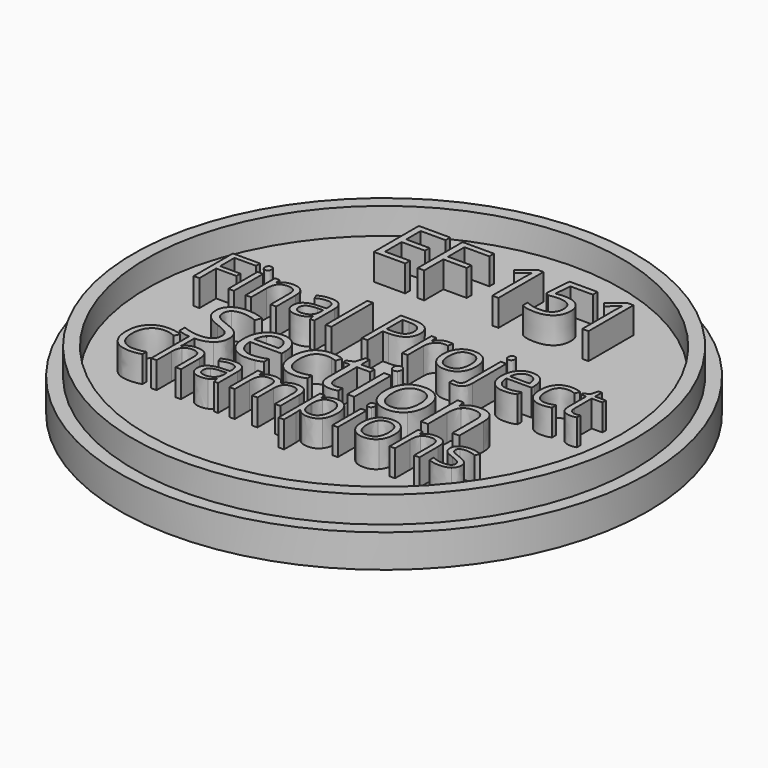
from build123d import *

# Parameters (mm, degrees)
F0_R           = 25.4
F1_DEPTH       = 3.175
F2_R           = 24.13
F2_R_2         = 22.86
F3_DEPTH       = 2.54
F4_TEXT_SIZE   = 7.5765898348
F4_TEXT_SIZE_2 = 6.592654649
F4_W           = 0.670269991
F4_H           = 4.4232653547
F4_W_2         = 0.5213210837
F4_H_2         = 3.4403173635
F5_DEPTH       = 2.54


# Not quite as in the source:
# - Text() gives the source's letters only with a copy of the font that has no kerning and outlines rounded to 1/6400 em; it was checked with that copy


with BuildPart() as f1:
    # F0 (on Top) → F1 (new body)
    with BuildSketch(Plane.XY):
        Circle(F0_R)
    extrude(amount=F1_DEPTH)

    # F2 (on face) → F3 (join)
    with BuildSketch(Plane.XY.offset(3.175)):
        Circle(F2_R)
        Circle(F2_R_2, mode=Mode.SUBTRACT)
    extrude(amount=F3_DEPTH)

    # F4 (on face) → F5 (join)
    with BuildSketch(Plane.XY.offset(3.175)):
        with Locations((-10.9458046269, 11.5243140608)):
            Text('EF 151', F4_TEXT_SIZE, font='Open Sans', text_align=(TextAlign.LEFT, TextAlign.BOTTOM))
        with Locations((-18.9641831386, 0)):
            Text('Final Project', F4_TEXT_SIZE_2, font='Open Sans', text_align=(TextAlign.LEFT, TextAlign.BOTTOM))
        with BuildLine():
            add(Edge.make_bspline(
                [(-9.8868052331, -6.2462335304), (-9.8868052331, -7.0249865257), (-10.4518208806, -7.4615014716)],
                knots=[0, 0, 0, 1, 1, 1], degree=2))
            add(Edge.make_bspline(
                [(-10.2355006041, -5.2621377055), (-9.8868052331, -5.6418282206), (-9.8868052331, -6.2462335304)],
                knots=[0, 0, 0, 1, 1, 1], degree=2))
            add(Edge.make_bspline(
                [(-11.5127588335, -4.55183232), (-10.5841959751, -4.8824471903), (-10.2355006041, -5.2621377055)],
                knots=[0, 0, 0, 1, 1, 1], degree=2))
            add(Edge.make_bspline(
                [(-12.334130152, -4.1908680378), (-12.0655055698, -4.3542382764), (-11.5127588335, -4.55183232)],
                knots=[0, 0, 0, 1, 1, 1], degree=2))
            add(Edge.make_bspline(
                [(-12.7157578636, -3.8311952199), (-12.6027547341, -4.0274977991), (-12.334130152, -4.1908680378)],
                knots=[0, 0, 0, 1, 1, 1], degree=2))
            add(Edge.make_bspline(
                [(-12.8287609931, -3.3288155927), (-12.8287609931, -3.6348926406), (-12.7157578636, -3.8311952199)],
                knots=[0, 0, 0, 1, 1, 1], degree=2))
            add(Edge.make_bspline(
                [(-12.522038213, -2.6792090312), (-12.8287609931, -2.9129640762), (-12.8287609931, -3.3288155927)],
                knots=[0, 0, 0, 1, 1, 1], degree=2))
            add(Edge.make_bspline(
                [(-11.6703174827, -2.4454539861), (-12.2153154329, -2.4454539861), (-12.522038213, -2.6792090312)],
                knots=[0, 0, 0, 1, 1, 1], degree=2))
            add(Edge.make_bspline(
                [(-10.2497067118, -2.751531034), (-10.9806755266, -2.4454539861), (-11.6703174827, -2.4454539861)],
                knots=[0, 0, 0, 1, 1, 1], degree=2))
            Line((-10.2497067118, -2.751531034), (-10.0353236318, -2.1548745103))
            add(Edge.make_bspline(
                [(-11.6535284463, -1.832008426), (-10.7740412327, -1.832008426), (-10.0353236318, -2.1548745103)],
                knots=[0, 0, 0, 1, 1, 1], degree=2))
            add(Edge.make_bspline(
                [(-13.0102117325, -2.2355910313), (-12.4981461228, -1.832008426), (-11.6535284463, -1.832008426)],
                knots=[0, 0, 0, 1, 1, 1], degree=2))
            add(Edge.make_bspline(
                [(-13.5222773421, -3.3210668067), (-13.5222773421, -2.6391736367), (-13.0102117325, -2.2355910313)],
                knots=[0, 0, 0, 1, 1, 1], degree=2))
            add(Edge.make_bspline(
                [(-13.1690618459, -4.3742559737), (-13.5222773421, -3.9706733683), (-13.5222773421, -3.3210668067)],
                knots=[0, 0, 0, 1, 1, 1], degree=2))
            add(Edge.make_bspline(
                [(-11.993183567, -5.0722924479), (-12.8158463497, -4.777838579), (-13.1690618459, -4.3742559737)],
                knots=[0, 0, 0, 1, 1, 1], degree=2))
            add(Edge.make_bspline(
                [(-11.1156335499, -5.4474628378), (-11.4042758292, -5.2815096705), (-11.993183567, -5.0722924479)],
                knots=[0, 0, 0, 1, 1, 1], degree=2))
            add(Edge.make_bspline(
                [(-10.7036564263, -5.8090728522), (-10.8269912705, -5.6134160052), (-11.1156335499, -5.4474628378)],
                knots=[0, 0, 0, 1, 1, 1], degree=2))
            add(Edge.make_bspline(
                [(-10.5803215821, -6.3108067472), (-10.5803215821, -6.0047296993), (-10.7036564263, -5.8090728522)],
                knots=[0, 0, 0, 1, 1, 1], degree=2))
            add(Edge.make_bspline(
                [(-10.9277254888, -7.0359639725), (-10.5803215821, -6.7757339086), (-10.5803215821, -6.3108067472)],
                knots=[0, 0, 0, 1, 1, 1], degree=2))
            add(Edge.make_bspline(
                [(-11.9608969585, -7.2961940365), (-11.2751293955, -7.2961940365), (-10.9277254888, -7.0359639725)],
                knots=[0, 0, 0, 1, 1, 1], degree=2))
            add(Edge.make_bspline(
                [(-12.8080975637, -7.2070829972), (-12.3806228681, -7.2961940365), (-11.9608969585, -7.2961940365)],
                knots=[0, 0, 0, 1, 1, 1], degree=2))
            add(Edge.make_bspline(
                [(-13.5997652024, -6.9655791662), (-13.2355722593, -7.1179719579), (-12.8080975637, -7.2070829972)],
                knots=[0, 0, 0, 1, 1, 1], degree=2))
            Line((-13.5997652024, -6.9655791662), (-13.5997652024, -7.6268089068))
            add(Edge.make_bspline(
                [(-12.4609801616, -7.8823944824), (-13.1698642161, -7.832925818), (-13.5997652024, -7.6268089068)],
                knots=[0.2400029386, 0.2400029386, 0.2400029386, 1, 1, 1], degree=2))
            Line((-12.4609801616, -7.8823944824), (-12.4609801616, -7.5605137475))
            Line((-12.4609801616, -7.5605137475), (-11.9396590779, -7.5605137475))
            Line((-11.9396590779, -7.5605137475), (-11.9396590779, -7.8977702507))
            add(Edge.make_bspline(
                [(-10.4518208806, -7.4615014716), (-11.0034188994, -7.887650341), (-11.9396590779, -7.8977702507)],
                knots=[0, 0, 0, 0.9762526424, 0.9762526424, 0.9762526424], degree=2))
        make_face()
        with BuildLine():
            Line((-11.9396590779, -9.0390968596), (-11.9396590779, -7.8977702507))
            add(Edge.make_bspline(
                [(-11.9396590779, -7.8977702507), (-11.9624331318, -7.8980164176), (-11.9854347809, -7.8980164176)],
                knots=[0.9762526424, 0.9762526424, 0.9762526424, 1, 1, 1], degree=2))
            add(Edge.make_bspline(
                [(-11.9854347809, -7.8980164176), (-12.2371184326, -7.8980164176), (-12.4609801616, -7.8823944824)],
                knots=[0, 0, 0, 0.2400029386, 0.2400029386, 0.2400029386], degree=2))
            Line((-12.4609801616, -7.8823944824), (-12.4609801616, -12.4452621676))
            Line((-12.4609801616, -12.4452621676), (-11.9396590779, -12.4452621676))
            Line((-11.9396590779, -12.4452621676), (-11.9396590779, -10.6462524163))
            add(Edge.make_bspline(
                [(-11.6900477305, -9.6799501379), (-11.9396590779, -9.9752649714), (-11.9396590779, -10.6462524163)],
                knots=[0, 0, 0, 1, 1, 1], degree=2))
            add(Edge.make_bspline(
                [(-10.8980213827, -9.3846353043), (-11.4404363831, -9.3846353043), (-11.6900477305, -9.6799501379)],
                knots=[0, 0, 0, 1, 1, 1], degree=2))
            add(Edge.make_bspline(
                [(-10.2978492295, -9.5920588184), (-10.4892011879, -9.3846353043), (-10.8980213827, -9.3846353043)],
                knots=[0, 0, 0, 1, 1, 1], degree=2))
            add(Edge.make_bspline(
                [(-10.106497271, -10.2193517216), (-10.106497271, -9.7994823324), (-10.2978492295, -9.5920588184)],
                knots=[0, 0, 0, 1, 1, 1], degree=2))
            Line((-10.106497271, -10.2193517216), (-10.106497271, -12.4452621676))
            Line((-10.106497271, -12.4452621676), (-9.5851761873, -12.4452621676))
            Line((-9.5851761873, -12.4452621676), (-9.5851761873, -10.2012712216))
            add(Edge.make_bspline(
                [(-9.9010827014, -9.2485293181), (-9.5851761873, -9.5483642767), (-9.5851761873, -10.2012712216)],
                knots=[0, 0, 0, 1, 1, 1], degree=2))
            add(Edge.make_bspline(
                [(-10.8477977715, -8.9486943596), (-10.2169892155, -8.9486943596), (-9.9010827014, -9.2485293181)],
                knots=[0, 0, 0, 1, 1, 1], degree=2))
            add(Edge.make_bspline(
                [(-11.4956823553, -9.0913294152), (-11.2114167162, -8.9486943596), (-10.8477977715, -8.9486943596)],
                knots=[0, 0, 0, 1, 1, 1], degree=2))
            add(Edge.make_bspline(
                [(-11.9336322445, -9.48206911), (-11.7799479944, -9.2339644709), (-11.4956823553, -9.0913294152)],
                knots=[0, 0, 0, 1, 1, 1], degree=2))
            Line((-11.9336322445, -9.48206911), (-11.9647708834, -9.48206911))
            add(Edge.make_bspline(
                [(-11.9396590779, -9.0390968596), (-11.9396590779, -9.3062864709), (-11.9647708834, -9.48206911)],
                knots=[0, 0, 0, 1, 1, 1], degree=2))
        make_face()
        with BuildLine():
            add(Edge.make_bspline(
                [(-11.9396590779, -7.8977702507), (-11.9624331318, -7.8980164176), (-11.9854347809, -7.8980164176)],
                knots=[0.9762526424, 0.9762526424, 0.9762526424, 1, 1, 1], degree=2))
            Line((-11.9396590779, -7.8977702507), (-11.9396590779, -7.5605137475))
            Line((-11.9396590779, -7.5605137475), (-12.4609801616, -7.5605137475))
            Line((-12.4609801616, -7.5605137475), (-12.4609801616, -7.8823944824))
            add(Edge.make_bspline(
                [(-11.9854347809, -7.8980164176), (-12.2371184326, -7.8980164176), (-12.4609801616, -7.8823944824)],
                knots=[0, 0, 0, 0.2400029386, 0.2400029386, 0.2400029386], degree=2))
        make_face()
        with BuildLine():
            add(Edge.make_bspline(
                [(-6.9112714003, -7.8980164176), (-7.8914928322, -7.8980164176), (-8.4590914083, -7.3000684295)],
                knots=[0, 0, 0, 1, 1, 1], degree=2))
            add(Edge.make_bspline(
                [(-6.1467245127, -7.8308602721), (-6.4631332753, -7.8980164176), (-6.9112714003, -7.8980164176)],
                knots=[0, 0, 0, 1, 1, 1], degree=2))
            add(Edge.make_bspline(
                [(-5.4751630574, -7.6113113347), (-5.8303157501, -7.7637041265), (-6.1467245127, -7.8308602721)],
                knots=[0, 0, 0, 1, 1, 1], degree=2))
            Line((-5.4751630574, -7.6113113347), (-5.4751630574, -7.0133633466))
            add(Edge.make_bspline(
                [(-6.8867335779, -7.3116916085), (-6.1725537994, -7.3116916085), (-5.4751630574, -7.0133633466)],
                knots=[0, 0, 0, 1, 1, 1], degree=2))
            add(Edge.make_bspline(
                [(-7.9379855483, -6.9081090032), (-7.5647523549, -7.3116916085), (-6.8867335779, -7.3116916085)],
                knots=[0, 0, 0, 1, 1, 1], degree=2))
            add(Edge.make_bspline(
                [(-8.3318821711, -5.7257734025), (-8.3112187417, -6.5045263978), (-7.9379855483, -6.9081090032)],
                knots=[0, 0, 0, 1, 1, 1], degree=2))
            Line((-8.3318821711, -5.7257734025), (-5.2853177998, -5.7257734025))
            Line((-5.2853177998, -5.7257734025), (-5.2853177998, -5.3021730999))
            add(Edge.make_bspline(
                [(-5.7696169262, -3.8589617031), (-5.2853177998, -4.4058968499), (-5.2853177998, -5.3021730999)],
                knots=[0, 0, 0, 1, 1, 1], degree=2))
            add(Edge.make_bspline(
                [(-7.0843276214, -3.3120265564), (-6.2539160527, -3.3120265564), (-5.7696169262, -3.8589617031)],
                knots=[0, 0, 0, 1, 1, 1], degree=2))
            add(Edge.make_bspline(
                [(-8.499772535, -3.9416154207), (-7.9728550854, -3.3120265564), (-7.0843276214, -3.3120265564)],
                knots=[0, 0, 0, 1, 1, 1], degree=2))
            add(Edge.make_bspline(
                [(-9.0266899845, -5.6418282206), (-9.0266899845, -4.5712042851), (-8.499772535, -3.9416154207)],
                knots=[0, 0, 0, 1, 1, 1], degree=2))
            add(Edge.make_bspline(
                [(-8.4590914083, -7.3000684295), (-9.0266899845, -6.7021204414), (-9.0266899845, -5.6418282206)],
                knots=[0, 0, 0, 1, 1, 1], degree=2))
        make_face()
        with BuildLine():
            add(Edge.make_bspline(
                [(-7.0933678718, -3.873813543), (-7.6254511787, -3.873813543), (-7.9425056735, -4.2205717175)],
                knots=[0, 0, 0, 1, 1, 1], degree=2))
            add(Edge.make_bspline(
                [(-6.2855569289, -4.210885735), (-6.5677418866, -3.873813543), (-7.0933678718, -3.873813543)],
                knots=[0, 0, 0, 1, 1, 1], degree=2))
            add(Edge.make_bspline(
                [(-6.0033719712, -5.1807754522), (-6.0033719712, -4.547957927), (-6.2855569289, -4.210885735)],
                knots=[0, 0, 0, 1, 1, 1], degree=2))
            Line((-6.0033719712, -5.1807754522), (-8.3163845991, -5.1807754522))
            add(Edge.make_bspline(
                [(-7.9425056735, -4.2205717175), (-8.2595601682, -4.5673298921), (-8.3163845991, -5.1807754522)],
                knots=[0, 0, 0, 1, 1, 1], degree=2))
        make_face(mode=Mode.SUBTRACT)
        with BuildLine():
            add(Edge.make_bspline(
                [(-2.3743571839, -7.8980164176), (-3.3352066507, -7.8980164176), (-3.8621241003, -7.3065257512)],
                knots=[0, 0, 0, 1, 1, 1], degree=2))
            add(Edge.make_bspline(
                [(-1.2572405322, -7.6668443012), (-1.7002127999, -7.8980164176), (-2.3743571839, -7.8980164176)],
                knots=[0, 0, 0, 1, 1, 1], degree=2))
            Line((-1.2572405322, -7.6668443012), (-1.2572405322, -7.0740621705))
            add(Edge.make_bspline(
                [(-2.3911462202, -7.3116916085), (-1.8383994839, -7.3116916085), (-1.2572405322, -7.0740621705)],
                knots=[0, 0, 0, 1, 1, 1], degree=2))
            add(Edge.make_bspline(
                [(-3.3655560626, -6.8758223947), (-3.0368783888, -7.3116916085), (-2.3911462202, -7.3116916085)],
                knots=[0, 0, 0, 1, 1, 1], degree=2))
            add(Edge.make_bspline(
                [(-3.6942337364, -5.6250391842), (-3.6942337364, -6.4399531809), (-3.3655560626, -6.8758223947)],
                knots=[0, 0, 0, 1, 1, 1], degree=2))
            add(Edge.make_bspline(
                [(-2.3459449684, -3.9061001515), (-3.6942337364, -3.9061001515), (-3.6942337364, -5.6250391842)],
                knots=[0, 0, 0, 1, 1, 1], degree=2))
            add(Edge.make_bspline(
                [(-1.8823092714, -3.9642160466), (-2.1444765318, -3.9061001515), (-2.3459449684, -3.9061001515)],
                knots=[0, 0, 0, 1, 1, 1], degree=2))
            add(Edge.make_bspline(
                [(-1.398010145, -4.1114429811), (-1.620142011, -4.0223319418), (-1.8823092714, -3.9642160466)],
                knots=[0, 0, 0, 1, 1, 1], degree=2))
            Line((-1.398010145, -4.1114429811), (-1.1926673154, -3.5431986727))
            add(Edge.make_bspline(
                [(-1.6924640138, -3.3811198984), (-1.3734723226, -3.4502132404), (-1.1926673154, -3.5431986727)],
                knots=[0, 0, 0, 1, 1, 1], degree=2))
            add(Edge.make_bspline(
                [(-2.3304473964, -3.3120265564), (-2.0114557051, -3.3120265564), (-1.6924640138, -3.3811198984)],
                knots=[0, 0, 0, 1, 1, 1], degree=2))
            add(Edge.make_bspline(
                [(-3.8537295821, -3.9177233305), (-3.3184176143, -3.3120265564), (-2.3304473964, -3.3120265564)],
                knots=[0, 0, 0, 1, 1, 1], degree=2))
            add(Edge.make_bspline(
                [(-4.3890415498, -5.6327879702), (-4.3890415498, -4.5234201046), (-3.8537295821, -3.9177233305)],
                knots=[0, 0, 0, 1, 1, 1], degree=2))
            add(Edge.make_bspline(
                [(-3.8621241003, -7.3065257512), (-4.3890415498, -6.7150350848), (-4.3890415498, -5.6327879702)],
                knots=[0, 0, 0, 1, 1, 1], degree=2))
        make_face()
        with BuildLine():
            add(Edge.make_bspline(
                [(1.2210795308, -7.3439782169), (1.3993016093, -7.3439782169), (1.5646090445, -7.3181489302)],
                knots=[0, 0, 0, 1, 1, 1], degree=2))
            add(Edge.make_bspline(
                [(0.7006194029, -7.1302408691), (0.8904646605, -7.3439782169), (1.2210795308, -7.3439782169)],
                knots=[0, 0, 0, 1, 1, 1], degree=2))
            add(Edge.make_bspline(
                [(0.5107741453, -6.5174410412), (0.5107741453, -6.9165035213), (0.7006194029, -7.1302408691)],
                knots=[0, 0, 0, 1, 1, 1], degree=2))
            Line((0.5107741453, -6.5174410412), (0.5107741453, -3.9138489375))
            Line((0.5107741453, -3.9138489375), (1.7944896965, -3.9138489375))
            Line((1.7944896965, -3.9138489375), (1.7944896965, -3.3933888096))
            Line((1.7944896965, -3.3933888096), (0.5107741453, -3.3933888096))
            Line((0.5107741453, -3.3933888096), (0.5107741453, -2.3679661259))
            Line((0.5107741453, -2.3679661259), (0.1233348442, -2.3679661259))
            Line((0.1233348442, -2.3679661259), (-0.1582043813, -3.3120265564))
            Line((-0.1582043813, -3.3120265564), (-0.7923133708, -3.5909828532))
            Line((-0.7923133708, -3.5909828532), (-0.7923133708, -3.9138489375))
            Line((-0.7923133708, -3.9138489375), (-0.1582043813, -3.9138489375))
            Line((-0.1582043813, -3.9138489375), (-0.1582043813, -6.5458532566))
            add(Edge.make_bspline(
                [(1.1242197055, -7.8980164176), (-0.1582043813, -7.8980164176), (-0.1582043813, -6.5458532566)],
                knots=[0, 0, 0, 1, 1, 1], degree=2))
            add(Edge.make_bspline(
                [(1.5064931493, -7.8631468805), (1.294692998, -7.8980164176), (1.1242197055, -7.8980164176)],
                knots=[0, 0, 0, 1, 1, 1], degree=2))
            add(Edge.make_bspline(
                [(1.8267763049, -7.7766187699), (1.7182933006, -7.8282773434), (1.5064931493, -7.8631468805)],
                knots=[0, 0, 0, 1, 1, 1], degree=2))
            Line((1.8267763049, -7.7766187699), (1.8267763049, -7.263907428))
            add(Edge.make_bspline(
                [(1.5646090445, -7.3181489302), (1.7299164796, -7.2923196435), (1.8267763049, -7.263907428)],
                knots=[0, 0, 0, 1, 1, 1], degree=2))
        make_face()
        with Locations((3.045272907, -5.605021487)):
            Rectangle(F4_W, F4_H)
        with BuildLine():
            add(Edge.make_bspline(
                [(2.6533134807, -2.1949099047), (2.6533134807, -1.9650292527), (2.7663166102, -1.8578377127)],
                knots=[0, 0, 0, 1, 1, 1], degree=2))
            add(Edge.make_bspline(
                [(2.7663166102, -2.5319820967), (2.6533134807, -2.4209161637), (2.6533134807, -2.1949099047)],
                knots=[0, 0, 0, 1, 1, 1], degree=2))
            add(Edge.make_bspline(
                [(3.0497930322, -2.6430480297), (2.8793197397, -2.6430480297), (2.7663166102, -2.5319820967)],
                knots=[0, 0, 0, 1, 1, 1], degree=2))
            add(Edge.make_bspline(
                [(3.3281035968, -2.5319820967), (3.2112260743, -2.6430480297), (3.0497930322, -2.6430480297)],
                knots=[0, 0, 0, 1, 1, 1], degree=2))
            add(Edge.make_bspline(
                [(3.4449811194, -2.1949099047), (3.4449811194, -2.4209161637), (3.3281035968, -2.5319820967)],
                knots=[0, 0, 0, 1, 1, 1], degree=2))
            add(Edge.make_bspline(
                [(3.3281035968, -1.8597749092), (3.4449811194, -1.9689036457), (3.4449811194, -2.1949099047)],
                knots=[0, 0, 0, 1, 1, 1], degree=2))
            add(Edge.make_bspline(
                [(3.0497930322, -1.7506461727), (3.2112260743, -1.7506461727), (3.3281035968, -1.8597749092)],
                knots=[0, 0, 0, 1, 1, 1], degree=2))
            add(Edge.make_bspline(
                [(2.7663166102, -1.8578377127), (2.8793197397, -1.7506461727), (3.0497930322, -1.7506461727)],
                knots=[0, 0, 0, 1, 1, 1], degree=2))
        make_face()
        with BuildLine():
            add(Edge.make_bspline(
                [(8.618587254, -5.6005013618), (8.618587254, -6.6827484763), (8.0742350359, -7.290382447)],
                knots=[0, 0, 0, 1, 1, 1], degree=2))
            add(Edge.make_bspline(
                [(8.0716521072, -3.9299922417), (8.618587254, -4.547957927), (8.618587254, -5.6005013618)],
                knots=[0, 0, 0, 1, 1, 1], degree=2))
            add(Edge.make_bspline(
                [(6.5974455663, -3.3120265564), (7.5247169604, -3.3120265564), (8.0716521072, -3.9299922417)],
                knots=[0, 0, 0, 1, 1, 1], degree=2))
            add(Edge.make_bspline(
                [(5.0954725422, -3.915786134), (5.6365960995, -3.3120265564), (6.5974455663, -3.3120265564)],
                knots=[0, 0, 0, 1, 1, 1], degree=2))
            add(Edge.make_bspline(
                [(4.554348985, -5.6005013618), (4.554348985, -4.5195457116), (5.0954725422, -3.915786134)],
                knots=[0, 0, 0, 1, 1, 1], degree=2))
            add(Edge.make_bspline(
                [(4.8048930664, -6.8196436961), (4.554348985, -6.2991835682), (4.554348985, -5.6005013618)],
                knots=[0, 0, 0, 1, 1, 1], degree=2))
            add(Edge.make_bspline(
                [(5.5151984518, -7.6190601208), (5.0554371478, -7.3401038239), (4.8048930664, -6.8196436961)],
                knots=[0, 0, 0, 1, 1, 1], degree=2))
            add(Edge.make_bspline(
                [(6.5690333509, -7.8980164176), (5.9749597558, -7.8980164176), (5.5151984518, -7.6190601208)],
                knots=[0, 0, 0, 1, 1, 1], degree=2))
            add(Edge.make_bspline(
                [(8.0742350359, -7.290382447), (7.5298828178, -7.8980164176), (6.5690333509, -7.8980164176)],
                knots=[0, 0, 0, 1, 1, 1], degree=2))
        make_face()
        with BuildLine():
            add(Edge.make_bspline(
                [(5.2491567984, -5.6005013618), (5.2491567984, -6.4489934313), (5.5881661869, -6.8926114311)],
                knots=[0, 0, 0, 1, 1, 1], degree=2))
            add(Edge.make_bspline(
                [(5.5842917938, -4.3135571498), (5.2491567984, -4.7455519706), (5.2491567984, -5.6005013618)],
                knots=[0, 0, 0, 1, 1, 1], degree=2))
            add(Edge.make_bspline(
                [(6.5767821369, -3.881562329), (5.9194267893, -3.881562329), (5.5842917938, -4.3135571498)],
                knots=[0, 0, 0, 1, 1, 1], degree=2))
            add(Edge.make_bspline(
                [(7.5841243199, -4.3193687393), (7.2431777349, -3.881562329), (6.5767821369, -3.881562329)],
                knots=[0, 0, 0, 1, 1, 1], degree=2))
            add(Edge.make_bspline(
                [(7.9250709049, -5.6005013618), (7.9250709049, -4.7571751496), (7.5841243199, -4.3193687393)],
                knots=[0, 0, 0, 1, 1, 1], degree=2))
            add(Edge.make_bspline(
                [(7.5841243199, -6.8945486276), (7.9250709049, -6.4528678243), (7.9250709049, -5.6005013618)],
                knots=[0, 0, 0, 1, 1, 1], degree=2))
            add(Edge.make_bspline(
                [(6.584530923, -7.3362294309), (7.2431777349, -7.3362294309), (7.5841243199, -6.8945486276)],
                knots=[0, 0, 0, 1, 1, 1], degree=2))
            add(Edge.make_bspline(
                [(5.5881661869, -6.8926114311), (5.9271755754, -7.3362294309), (6.584530923, -7.3362294309)],
                knots=[0, 0, 0, 1, 1, 1], degree=2))
        make_face(mode=Mode.SUBTRACT)
        with BuildLine():
            Line((12.8210122071, -4.9547691932), (12.8210122071, -7.8166541643))
            Line((12.8210122071, -7.8166541643), (13.491282198, -7.8166541643))
            Line((13.491282198, -7.8166541643), (13.491282198, -4.9315228351))
            add(Edge.make_bspline(
                [(13.0876995927, -3.697528661), (13.491282198, -4.0830307656), (13.491282198, -4.9315228351)],
                knots=[0, 0, 0, 1, 1, 1], degree=2))
            add(Edge.make_bspline(
                [(11.8847005626, -3.3120265564), (12.6841169873, -3.3120265564), (13.0876995927, -3.697528661)],
                knots=[0, 0, 0, 1, 1, 1], degree=2))
            add(Edge.make_bspline(
                [(11.0575176547, -3.4921858314), (11.4288136516, -3.3120265564), (11.8847005626, -3.3120265564)],
                knots=[0, 0, 0, 1, 1, 1], degree=2))
            add(Edge.make_bspline(
                [(10.4795873638, -3.9990855837), (10.6862216578, -3.6723451064), (11.0575176547, -3.4921858314)],
                knots=[0, 0, 0, 1, 1, 1], degree=2))
            Line((10.4795873638, -3.9990855837), (10.4473007554, -3.9990855837))
            Line((10.4473007554, -3.9990855837), (10.3388177511, -3.3933888096))
            Line((10.3388177511, -3.3933888096), (9.7938198008, -3.3933888096))
            Line((9.7938198008, -3.3933888096), (9.7938198008, -7.8166541643))
            Line((9.7938198008, -7.8166541643), (10.4640897918, -7.8166541643))
            Line((10.4640897918, -7.8166541643), (10.4640897918, -5.4958927505))
            add(Edge.make_bspline(
                [(10.7869558761, -4.256732719), (10.4640897918, -4.6319031089), (10.4640897918, -5.4958927505)],
                knots=[0, 0, 0, 1, 1, 1], degree=2))
            add(Edge.make_bspline(
                [(11.8033383094, -3.881562329), (11.1098219603, -3.881562329), (10.7869558761, -4.256732719)],
                knots=[0, 0, 0, 1, 1, 1], degree=2))
            add(Edge.make_bspline(
                [(12.5749882508, -4.1482497147), (12.3289642946, -3.881562329), (11.8033383094, -3.881562329)],
                knots=[0, 0, 0, 1, 1, 1], degree=2))
            add(Edge.make_bspline(
                [(12.8210122071, -4.9547691932), (12.8210122071, -4.4149371003), (12.5749882508, -4.1482497147)],
                knots=[0, 0, 0, 1, 1, 1], degree=2))
        make_face()
        with BuildLine():
            add(Edge.make_bspline(
                [(-14.4739424963, -8.2676621924), (-15.2303100802, -8.2676621924), (-15.6682599694, -8.7714050122)],
                knots=[0, 0, 0, 1, 1, 1], degree=2))
            add(Edge.make_bspline(
                [(-13.4313003289, -8.5117489426), (-13.9526214126, -8.2676621924), (-14.4739424963, -8.2676621924)],
                knots=[0, 0, 0, 1, 1, 1], degree=2))
            Line((-13.4313003289, -8.5117489426), (-13.2052940787, -8.053709609))
            add(Edge.make_bspline(
                [(-14.4669111907, -7.7905378865), (-13.7457001347, -7.7905378865), (-13.2052940787, -8.053709609)],
                knots=[0, 0, 0, 1, 1, 1], degree=2))
            add(Edge.make_bspline(
                [(-15.6456593443, -8.0793236506), (-15.1449299412, -7.7905378865), (-14.4669111907, -7.7905378865)],
                knots=[0, 0, 0, 1, 1, 1], degree=2))
            add(Edge.make_bspline(
                [(-16.4115694143, -8.9014841651), (-16.1463887475, -8.3681094147), (-15.6456593443, -8.0793236506)],
                knots=[0, 0, 0, 1, 1, 1], degree=2))
            add(Edge.make_bspline(
                [(-16.6767500812, -10.1440163049), (-16.6767500812, -9.4348589155), (-16.4115694143, -8.9014841651)],
                knots=[0, 0, 0, 1, 1, 1], degree=2))
            add(Edge.make_bspline(
                [(-16.1257970669, -11.892802445), (-16.6767500812, -11.2770609723), (-16.6767500812, -10.1440163049)],
                knots=[0, 0, 0, 1, 1, 1], degree=2))
            add(Edge.make_bspline(
                [(-14.5613315797, -12.5085439176), (-15.5748440526, -12.5085439176), (-16.1257970669, -11.892802445)],
                knots=[0, 0, 0, 1, 1, 1], degree=2))
            add(Edge.make_bspline(
                [(-13.3840901344, -12.3287433897), (-13.8612144403, -12.5085439176), (-14.5613315797, -12.5085439176)],
                knots=[0, 0, 0, 1, 1, 1], degree=2))
            Line((-13.3840901344, -12.3287433897), (-13.3840901344, -11.8616638061))
            add(Edge.make_bspline(
                [(-14.4799693296, -12.0344330284), (-13.9998316071, -12.0344330284), (-13.3840901344, -11.8616638061)],
                knots=[0, 0, 0, 1, 1, 1], degree=2))
            add(Edge.make_bspline(
                [(-15.6838292888, -11.5427438753), (-15.2614487191, -12.0344330284), (-14.4799693296, -12.0344330284)],
                knots=[0, 0, 0, 1, 1, 1], degree=2))
            add(Edge.make_bspline(
                [(-16.1062098586, -10.1510476104), (-16.1062098586, -11.0510547222), (-15.6838292888, -11.5427438753)],
                knots=[0, 0, 0, 1, 1, 1], degree=2))
            add(Edge.make_bspline(
                [(-15.6682599694, -8.7714050122), (-16.1062098586, -9.275147832), (-16.1062098586, -10.1510476104)],
                knots=[0, 0, 0, 1, 1, 1], degree=2))
        make_face()
        with BuildLine():
            Line((-6.5034554074, -11.9550797228), (-6.3999947684, -12.4452621676))
            Line((-6.3999947684, -12.4452621676), (-6.0132729626, -12.4452621676))
            Line((-6.0132729626, -12.4452621676), (-6.0132729626, -10.0968061104))
            add(Edge.make_bspline(
                [(-6.3100945044, -9.2214085681), (-6.0132729626, -9.4941227766), (-6.0132729626, -10.0968061104)],
                knots=[0, 0, 0, 1, 1, 1], degree=2))
            add(Edge.make_bspline(
                [(-7.2216530468, -8.9486943596), (-6.6069160463, -8.9486943596), (-6.3100945044, -9.2214085681)],
                knots=[0, 0, 0, 1, 1, 1], degree=2))
            add(Edge.make_bspline(
                [(-7.8298609777, -9.027043193), (-7.5270126025, -8.9486943596), (-7.2216530468, -8.9486943596)],
                knots=[0, 0, 0, 1, 1, 1], degree=2))
            add(Edge.make_bspline(
                [(-8.3868408253, -9.2430047209), (-8.1327093529, -9.1053920264), (-7.8298609777, -9.027043193)],
                knots=[0, 0, 0, 1, 1, 1], degree=2))
            Line((-8.3868408253, -9.2430047209), (-8.2261252697, -9.6417801934))
            add(Edge.make_bspline(
                [(-7.2537961579, -9.378608471), (-7.6837102693, -9.378608471), (-8.2261252697, -9.6417801934)],
                knots=[0, 0, 0, 1, 1, 1], degree=2))
            add(Edge.make_bspline(
                [(-6.6963140742, -9.5714671378), (-6.8700877687, -9.378608471), (-7.2537961579, -9.378608471)],
                knots=[0, 0, 0, 1, 1, 1], degree=2))
            add(Edge.make_bspline(
                [(-6.5225403796, -10.1691281104), (-6.5225403796, -9.7643258046), (-6.6963140742, -9.5714671378)],
                knots=[0, 0, 0, 1, 1, 1], degree=2))
            Line((-6.5225403796, -10.1691281104), (-6.5225403796, -10.3830806939))
            Line((-6.5225403796, -10.3830806939), (-7.1061387411, -10.4021656662))
            add(Edge.make_bspline(
                [(-8.772558159, -11.4940269725), (-8.772558159, -10.4523892773), (-7.1061387411, -10.4021656662)],
                knots=[0, 0, 0, 1, 1, 1], degree=2))
            add(Edge.make_bspline(
                [(-8.4822656865, -12.244367723), (-8.772558159, -11.9801915284), (-8.772558159, -11.4940269725)],
                knots=[0, 0, 0, 1, 1, 1], degree=2))
            add(Edge.make_bspline(
                [(-7.6806968526, -12.5085439176), (-8.1919732141, -12.5085439176), (-8.4822656865, -12.244367723)],
                knots=[0, 0, 0, 1, 1, 1], degree=2))
            add(Edge.make_bspline(
                [(-7.0413502827, -12.3935318481), (-7.2969884635, -12.5085439176), (-7.6806968526, -12.5085439176)],
                knots=[0, 0, 0, 1, 1, 1], degree=2))
            add(Edge.make_bspline(
                [(-6.5285672129, -11.9550797228), (-6.785712102, -12.2785197786), (-7.0413502827, -12.3935318481)],
                knots=[0, 0, 0, 1, 1, 1], degree=2))
            Line((-6.5285672129, -11.9550797228), (-6.5034554074, -11.9550797228))
        make_face()
        with BuildLine():
            add(Edge.make_bspline(
                [(-7.5772362137, -12.077625334), (-7.0900671855, -12.077625334), (-6.8123306159, -11.8109379588)],
                knots=[0, 0, 0, 1, 1, 1], degree=2))
            add(Edge.make_bspline(
                [(-8.0553649918, -11.9304701534), (-7.8846047139, -12.077625334), (-7.5772362137, -12.077625334)],
                knots=[0, 0, 0, 1, 1, 1], degree=2))
            add(Edge.make_bspline(
                [(-8.2261252697, -11.5000538058), (-8.2261252697, -11.7833149727), (-8.0553649918, -11.9304701534)],
                knots=[0, 0, 0, 1, 1, 1], degree=2))
            add(Edge.make_bspline(
                [(-7.9519043528, -10.9681857638), (-8.2261252697, -11.1394482778), (-8.2261252697, -11.5000538058)],
                knots=[0, 0, 0, 1, 1, 1], degree=2))
            add(Edge.make_bspline(
                [(-7.05591513, -10.7748248609), (-7.677683436, -10.7969232498), (-7.9519043528, -10.9681857638)],
                knots=[0, 0, 0, 1, 1, 1], degree=2))
            Line((-7.05591513, -10.7748248609), (-6.5345940463, -10.7537309442))
            Line((-6.5345940463, -10.7537309442), (-6.5345940463, -11.0641128611))
            add(Edge.make_bspline(
                [(-6.8123306159, -11.8109379588), (-6.5345940463, -11.5442505836), (-6.5345940463, -11.0641128611)],
                knots=[0, 0, 0, 1, 1, 1], degree=2))
        make_face(mode=Mode.SUBTRACT)
        with BuildLine():
            Line((-0.5549709032, -10.2072980549), (-0.5549709032, -12.4452621676))
            Line((-0.5549709032, -12.4452621676), (-0.0346542917, -12.4452621676))
            Line((-0.0346542917, -12.4452621676), (-0.0346542917, -10.2012712216))
            add(Edge.make_bspline(
                [(-0.3249467641, -9.2414980126), (-0.0346542917, -9.5413329711), (-0.0346542917, -10.2012712216)],
                knots=[0, 0, 0, 1, 1, 1], degree=2))
            add(Edge.make_bspline(
                [(-1.1988375981, -8.941663054), (-0.6152392365, -8.941663054), (-0.3249467641, -9.2414980126)],
                knots=[0, 0, 0, 1, 1, 1], degree=2))
            add(Edge.make_bspline(
                [(-1.8643004458, -9.0988629569), (-1.572501265, -8.941663054), (-1.1988375981, -8.941663054)],
                knots=[0, 0, 0, 1, 1, 1], degree=2))
            add(Edge.make_bspline(
                [(-2.3097838766, -9.5262658878), (-2.1560996265, -9.2560628598), (-1.8643004458, -9.0988629569)],
                knots=[0, 0, 0, 1, 1, 1], degree=2))
            Line((-2.3097838766, -9.5262658878), (-2.3348956822, -9.5262658878))
            add(Edge.make_bspline(
                [(-3.3895915163, -8.941663054), (-2.5830003213, -8.941663054), (-2.3348956822, -9.5262658878)],
                knots=[0, 0, 0, 1, 1, 1], degree=2))
            add(Edge.make_bspline(
                [(-3.9907681417, -9.0832936375), (-3.7220718221, -8.941663054), (-3.3895915163, -8.941663054)],
                knots=[0, 0, 0, 1, 1, 1], degree=2))
            add(Edge.make_bspline(
                [(-4.4071218781, -9.4760422766), (-4.2594644613, -9.2249242209), (-3.9907681417, -9.0832936375)],
                knots=[0, 0, 0, 1, 1, 1], degree=2))
            Line((-4.4071218781, -9.4760422766), (-4.4322336837, -9.4760422766))
            Line((-4.4322336837, -9.4760422766), (-4.5166093504, -9.0049448041))
            Line((-4.5166093504, -9.0049448041), (-4.9404966285, -9.0049448041))
            Line((-4.9404966285, -9.0049448041), (-4.9404966285, -12.4452621676))
            Line((-4.9404966285, -12.4452621676), (-4.4191755448, -12.4452621676))
            Line((-4.4191755448, -12.4452621676), (-4.4191755448, -10.640225583))
            add(Edge.make_bspline(
                [(-4.1916625863, -9.6779411934), (-4.4191755448, -9.9712470825), (-4.4191755448, -10.640225583)],
                knots=[0, 0, 0, 1, 1, 1], degree=2))
            add(Edge.make_bspline(
                [(-3.4749716552, -9.3846353043), (-3.9641496278, -9.3846353043), (-4.1916625863, -9.6779411934)],
                knots=[0, 0, 0, 1, 1, 1], degree=2))
            add(Edge.make_bspline(
                [(-2.9255253493, -9.5900498739), (-3.1013079883, -9.3846353043), (-3.4749716552, -9.3846353043)],
                knots=[0, 0, 0, 1, 1, 1], degree=2))
            add(Edge.make_bspline(
                [(-2.7497427103, -10.2072980549), (-2.7497427103, -9.7954644435), (-2.9255253493, -9.5900498739)],
                knots=[0, 0, 0, 1, 1, 1], degree=2))
            Line((-2.7497427103, -10.2072980549), (-2.7497427103, -12.4452621676))
            Line((-2.7497427103, -12.4452621676), (-2.2284216266, -12.4452621676))
            Line((-2.2284216266, -12.4452621676), (-2.2284216266, -10.5237068051))
            add(Edge.make_bspline(
                [(-1.995886307, -9.6638785823), (-2.2284216266, -9.9431218603), (-2.2284216266, -10.5237068051)],
                knots=[0, 0, 0, 1, 1, 1], degree=2))
            add(Edge.make_bspline(
                [(-1.2771864315, -9.3846353043), (-1.7633509874, -9.3846353043), (-1.995886307, -9.6638785823)],
                knots=[0, 0, 0, 1, 1, 1], degree=2))
            add(Edge.make_bspline(
                [(-0.7307535422, -9.5900498739), (-0.9065361812, -9.3846353043), (-1.2771864315, -9.3846353043)],
                knots=[0, 0, 0, 1, 1, 1], degree=2))
            add(Edge.make_bspline(
                [(-0.5549709032, -10.2072980549), (-0.5549709032, -9.7954644435), (-0.7307535422, -9.5900498739)],
                knots=[0, 0, 0, 1, 1, 1], degree=2))
        make_face()
        with BuildLine():
            add(Edge.make_bspline(
                [(2.640255238, -12.5085439176), (2.3037570433, -12.5085439176), (2.0260204736, -12.3844915981)],
                knots=[0, 0, 0, 1, 1, 1], degree=2))
            add(Edge.make_bspline(
                [(3.690430947, -12.0389531534), (3.3122471551, -12.5085439176), (2.640255238, -12.5085439176)],
                knots=[0, 0, 0, 1, 1, 1], degree=2))
            add(Edge.make_bspline(
                [(4.068614739, -10.7215878331), (4.068614739, -11.5693623892), (3.690430947, -12.0389531534)],
                knots=[0, 0, 0, 1, 1, 1], degree=2))
            add(Edge.make_bspline(
                [(3.6964577804, -9.4097471099), (4.068614739, -9.8778311658), (4.068614739, -10.7215878331)],
                knots=[0, 0, 0, 1, 1, 1], degree=2))
            add(Edge.make_bspline(
                [(2.640255238, -8.941663054), (3.3243008218, -8.941663054), (3.6964577804, -9.4097471099)],
                knots=[0, 0, 0, 1, 1, 1], degree=2))
            add(Edge.make_bspline(
                [(2.0280294181, -9.0672220819), (2.2947167933, -8.941663054), (2.640255238, -8.941663054)],
                knots=[0, 0, 0, 1, 1, 1], degree=2))
            add(Edge.make_bspline(
                [(1.5604475983, -9.4760422766), (1.7613420429, -9.1927811098), (2.0280294181, -9.0672220819)],
                knots=[0, 0, 0, 1, 1, 1], degree=2))
            Line((1.5604475983, -9.4760422766), (1.5353357927, -9.4760422766))
            Line((1.5353357927, -9.4760422766), (1.4630137927, -9.0049448041))
            Line((1.4630137927, -9.0049448041), (1.0391265146, -9.0049448041))
            Line((1.0391265146, -9.0049448041), (1.0391265146, -13.9901404465))
            Line((1.0391265146, -13.9901404465), (1.5604475983, -13.9901404465))
            Line((1.5604475983, -13.9901404465), (1.5604475983, -12.5738346121))
            add(Edge.make_bspline(
                [(1.5222776538, -12.0022899173), (1.5604475983, -12.3036315842), (1.5604475983, -12.5738346121)],
                knots=[0, 0, 0, 1, 1, 1], degree=2))
            Line((1.5222776538, -12.0022899173), (1.5604475983, -12.0022899173))
            add(Edge.make_bspline(
                [(2.0260204736, -12.3844915981), (1.748283904, -12.2604392786), (1.5604475983, -12.0022899173)],
                knots=[0, 0, 0, 1, 1, 1], degree=2))
        make_face()
        with BuildLine():
            add(Edge.make_bspline(
                [(2.5649198213, -9.3846353043), (2.0375719042, -9.3846353043), (1.8020231679, -9.6764344851)],
                knots=[0, 0, 0, 1, 1, 1], degree=2))
            add(Edge.make_bspline(
                [(3.275583919, -9.7281648046), (3.0229591549, -9.3846353043), (2.5649198213, -9.3846353043)],
                knots=[0, 0, 0, 1, 1, 1], degree=2))
            add(Edge.make_bspline(
                [(3.528208683, -10.7155609997), (3.528208683, -10.0716943048), (3.275583919, -9.7281648046)],
                knots=[0, 0, 0, 1, 1, 1], degree=2))
            add(Edge.make_bspline(
                [(3.275583919, -11.7104907365), (3.528208683, -11.3493829724), (3.528208683, -10.7155609997)],
                knots=[0, 0, 0, 1, 1, 1], degree=2))
            add(Edge.make_bspline(
                [(2.5769734879, -12.0715985007), (3.0229591549, -12.0715985007), (3.275583919, -11.7104907365)],
                knots=[0, 0, 0, 1, 1, 1], degree=2))
            add(Edge.make_bspline(
                [(1.8020231679, -11.7592076393), (2.0435987375, -12.0715985007), (2.5769734879, -12.0715985007)],
                knots=[0, 0, 0, 1, 1, 1], degree=2))
            add(Edge.make_bspline(
                [(1.5604475983, -10.7215878331), (1.5604475983, -11.446816778), (1.8020231679, -11.7592076393)],
                knots=[0, 0, 0, 1, 1, 1], degree=2))
            Line((1.5604475983, -10.7215878331), (1.5604475983, -10.6060735274))
            add(Edge.make_bspline(
                [(1.8020231679, -9.6764344851), (1.5664744317, -9.9682336659), (1.5604475983, -10.6060735274)],
                knots=[0, 0, 0, 1, 1, 1], degree=2))
        make_face(mode=Mode.SUBTRACT)
        with Locations((5.2393271148, -10.7251034858)):
            Rectangle(F4_W_2, F4_H_2)
        with BuildLine():
            add(Edge.make_bspline(
                [(4.9344697951, -8.0727945812), (4.9344697951, -7.8939985255), (5.0223611146, -7.810627331)],
                knots=[0, 0, 0, 1, 1, 1], degree=2))
            add(Edge.make_bspline(
                [(5.0223611146, -8.3349618314), (4.9344697951, -8.2485772202), (4.9344697951, -8.0727945812)],
                knots=[0, 0, 0, 1, 1, 1], degree=2))
            add(Edge.make_bspline(
                [(5.2428427676, -8.4213464425), (5.1102524342, -8.4213464425), (5.0223611146, -8.3349618314)],
                knots=[0, 0, 0, 1, 1, 1], degree=2))
            add(Edge.make_bspline(
                [(5.4593065316, -8.3349618314), (5.3684017954, -8.4213464425), (5.2428427676, -8.4213464425)],
                knots=[0, 0, 0, 1, 1, 1], degree=2))
            add(Edge.make_bspline(
                [(5.5502112678, -8.0727945812), (5.5502112678, -8.2485772202), (5.4593065316, -8.3349618314)],
                knots=[0, 0, 0, 1, 1, 1], degree=2))
            add(Edge.make_bspline(
                [(5.4593065316, -7.8121340393), (5.5502112678, -7.8970119422), (5.5502112678, -8.0727945812)],
                knots=[0, 0, 0, 1, 1, 1], degree=2))
            add(Edge.make_bspline(
                [(5.2428427676, -7.7272561365), (5.3684017954, -7.7272561365), (5.4593065316, -7.8121340393)],
                knots=[0, 0, 0, 1, 1, 1], degree=2))
            add(Edge.make_bspline(
                [(5.0223611146, -7.810627331), (5.1102524342, -7.7272561365), (5.2428427676, -7.7272561365)],
                knots=[0, 0, 0, 1, 1, 1], degree=2))
        make_face()
        with BuildLine():
            add(Edge.make_bspline(
                [(9.5741269929, -10.7215878331), (9.5741269929, -11.5633355559), (9.1507419509, -12.0359397368)],
                knots=[0, 0, 0, 1, 1, 1], degree=2))
            add(Edge.make_bspline(
                [(9.1487330064, -9.4223030127), (9.5741269929, -9.9029429714), (9.5741269929, -10.7215878331)],
                knots=[0, 0, 0, 1, 1, 1], degree=2))
            add(Edge.make_bspline(
                [(8.002127964, -8.941663054), (8.72333902, -8.941663054), (9.1487330064, -9.4223030127)],
                knots=[0, 0, 0, 1, 1, 1], degree=2))
            add(Edge.make_bspline(
                [(6.8339267687, -9.4112538182), (7.2548006301, -8.941663054), (8.002127964, -8.941663054)],
                knots=[0, 0, 0, 1, 1, 1], degree=2))
            add(Edge.make_bspline(
                [(6.4130529073, -10.7215878331), (6.4130529073, -9.8808445825), (6.8339267687, -9.4112538182)],
                knots=[0, 0, 0, 1, 1, 1], degree=2))
            add(Edge.make_bspline(
                [(6.6079205185, -11.6698096115), (6.4130529073, -11.2650073057), (6.4130529073, -10.7215878331)],
                knots=[0, 0, 0, 1, 1, 1], degree=2))
            add(Edge.make_bspline(
                [(7.1603802412, -12.2915779175), (6.8027881298, -12.0746119173), (6.6079205185, -11.6698096115)],
                knots=[0, 0, 0, 1, 1, 1], degree=2))
            add(Edge.make_bspline(
                [(7.9800295751, -12.5085439176), (7.5179723525, -12.5085439176), (7.1603802412, -12.2915779175)],
                knots=[0, 0, 0, 1, 1, 1], degree=2))
            add(Edge.make_bspline(
                [(9.1507419509, -12.0359397368), (8.7273569089, -12.5085439176), (7.9800295751, -12.5085439176)],
                knots=[0, 0, 0, 1, 1, 1], degree=2))
        make_face()
        with BuildLine():
            add(Edge.make_bspline(
                [(6.9534589632, -10.7215878331), (6.9534589632, -11.3815260835), (7.2171329217, -11.7265622921)],
                knots=[0, 0, 0, 1, 1, 1], degree=2))
            add(Edge.make_bspline(
                [(7.2141195051, -9.7206312629), (6.9534589632, -10.0566272215), (6.9534589632, -10.7215878331)],
                knots=[0, 0, 0, 1, 1, 1], degree=2))
            add(Edge.make_bspline(
                [(7.9860564084, -9.3846353043), (7.4747800469, -9.3846353043), (7.2141195051, -9.7206312629)],
                knots=[0, 0, 0, 1, 1, 1], degree=2))
            add(Edge.make_bspline(
                [(8.7695447423, -9.7251513879), (8.5043640754, -9.3846353043), (7.9860564084, -9.3846353043)],
                knots=[0, 0, 0, 1, 1, 1], degree=2))
            add(Edge.make_bspline(
                [(9.0347254091, -10.7215878331), (9.0347254091, -10.0656674715), (8.7695447423, -9.7251513879)],
                knots=[0, 0, 0, 1, 1, 1], degree=2))
            add(Edge.make_bspline(
                [(8.7695447423, -11.7280690004), (9.0347254091, -11.3845395002), (9.0347254091, -10.7215878331)],
                knots=[0, 0, 0, 1, 1, 1], degree=2))
            add(Edge.make_bspline(
                [(7.9920832417, -12.0715985007), (8.5043640754, -12.0715985007), (8.7695447423, -11.7280690004)],
                knots=[0, 0, 0, 1, 1, 1], degree=2))
            add(Edge.make_bspline(
                [(7.2171329217, -11.7265622921), (7.4808068803, -12.0715985007), (7.9920832417, -12.0715985007)],
                knots=[0, 0, 0, 1, 1, 1], degree=2))
        make_face(mode=Mode.SUBTRACT)
        with BuildLine():
            Line((12.8426796063, -10.2193517216), (12.8426796063, -12.4452621676))
            Line((12.8426796063, -12.4452621676), (13.36400069, -12.4452621676))
            Line((13.36400069, -12.4452621676), (13.36400069, -10.2012712216))
            add(Edge.make_bspline(
                [(13.0501031203, -9.2414980126), (13.36400069, -9.5413329711), (13.36400069, -10.2012712216)],
                knots=[0, 0, 0, 1, 1, 1], degree=2))
            add(Edge.make_bspline(
                [(12.1144372446, -8.941663054), (12.7362055506, -8.941663054), (13.0501031203, -9.2414980126)],
                knots=[0, 0, 0, 1, 1, 1], degree=2))
            add(Edge.make_bspline(
                [(11.4710727859, -9.0817869291), (11.7598585499, -8.941663054), (12.1144372446, -8.941663054)],
                knots=[0, 0, 0, 1, 1, 1], degree=2))
            add(Edge.make_bspline(
                [(11.0215714661, -9.4760422766), (11.1822870218, -9.2219108042), (11.4710727859, -9.0817869291)],
                knots=[0, 0, 0, 1, 1, 1], degree=2))
            Line((11.0215714661, -9.4760422766), (10.9964596605, -9.4760422766))
            Line((10.9964596605, -9.4760422766), (10.9120839938, -9.0049448041))
            Line((10.9120839938, -9.0049448041), (10.4881967157, -9.0049448041))
            Line((10.4881967157, -9.0049448041), (10.4881967157, -12.4452621676))
            Line((10.4881967157, -12.4452621676), (11.0095177994, -12.4452621676))
            Line((11.0095177994, -12.4452621676), (11.0095177994, -10.640225583))
            add(Edge.make_bspline(
                [(11.2606358552, -9.6764344851), (11.0095177994, -9.9682336659), (11.0095177994, -10.640225583)],
                knots=[0, 0, 0, 1, 1, 1], degree=2))
            add(Edge.make_bspline(
                [(12.0511554946, -9.3846353043), (11.5117539109, -9.3846353043), (11.2606358552, -9.6764344851)],
                knots=[0, 0, 0, 1, 1, 1], degree=2))
            add(Edge.make_bspline(
                [(12.6513276478, -9.5920588184), (12.4599756893, -9.3846353043), (12.0511554946, -9.3846353043)],
                knots=[0, 0, 0, 1, 1, 1], degree=2))
            add(Edge.make_bspline(
                [(12.8426796063, -10.2193517216), (12.8426796063, -9.7994823324), (12.6513276478, -9.5920588184)],
                knots=[0, 0, 0, 1, 1, 1], degree=2))
        make_face()
        with BuildLine():
            add(Edge.make_bspline(
                [(16.6526427478, -11.5070851114), (16.6526427478, -11.9872228339), (16.2950506365, -12.2478833758)],
                knots=[0, 0, 0, 1, 1, 1], degree=2))
            add(Edge.make_bspline(
                [(16.4376856921, -10.9385538332), (16.6526427478, -11.1645600834), (16.6526427478, -11.5070851114)],
                knots=[0, 0, 0, 1, 1, 1], degree=2))
            add(Edge.make_bspline(
                [(15.6110050527, -10.4895547496), (16.2227286364, -10.712547583), (16.4376856921, -10.9385538332)],
                knots=[0, 0, 0, 1, 1, 1], degree=2))
            add(Edge.make_bspline(
                [(15.0083217189, -10.234921041), (15.1650193857, -10.3228123606), (15.6110050527, -10.4895547496)],
                knots=[0, 0, 0, 1, 1, 1], degree=2))
            add(Edge.make_bspline(
                [(14.7808087604, -10.050098152), (14.8516240521, -10.1470297215), (15.0083217189, -10.234921041)],
                knots=[0, 0, 0, 1, 1, 1], degree=2))
            add(Edge.make_bspline(
                [(14.7099934687, -9.8145494158), (14.7099934687, -9.9531665825), (14.7808087604, -10.050098152)],
                knots=[0, 0, 0, 1, 1, 1], degree=2))
            add(Edge.make_bspline(
                [(14.8983320105, -9.4946250127), (14.7099934687, -9.6106415545), (14.7099934687, -9.8145494158)],
                knots=[0, 0, 0, 1, 1, 1], degree=2))
            add(Edge.make_bspline(
                [(15.4573208025, -9.378608471), (15.0866705523, -9.378608471), (14.8983320105, -9.4946250127)],
                knots=[0, 0, 0, 1, 1, 1], degree=2))
            add(Edge.make_bspline(
                [(16.3954978588, -9.5915565823), (15.878194664, -9.378608471), (15.4573208025, -9.378608471)],
                knots=[0, 0, 0, 1, 1, 1], degree=2))
            Line((16.3954978588, -9.5915565823), (16.58132522, -9.1676693042))
            add(Edge.make_bspline(
                [(15.4944862748, -8.941663054), (16.0499594141, -8.941663054), (16.58132522, -9.1676693042)],
                knots=[0, 0, 0, 1, 1, 1], degree=2))
            add(Edge.make_bspline(
                [(14.5563092186, -9.1852475681), (14.8988342466, -8.941663054), (15.4944862748, -8.941663054)],
                knots=[0, 0, 0, 1, 1, 1], degree=2))
            add(Edge.make_bspline(
                [(14.2137841906, -9.8497059436), (14.2137841906, -9.4288320821), (14.5563092186, -9.1852475681)],
                knots=[0, 0, 0, 1, 1, 1], degree=2))
            add(Edge.make_bspline(
                [(14.3127247045, -10.2540060133), (14.2137841906, -10.0847524437), (14.2137841906, -9.8497059436)],
                knots=[0, 0, 0, 1, 1, 1], degree=2))
            add(Edge.make_bspline(
                [(14.6140663714, -10.5568543885), (14.4116652185, -10.4232595828), (14.3127247045, -10.2540060133)],
                knots=[0, 0, 0, 1, 1, 1], degree=2))
            add(Edge.make_bspline(
                [(15.2966052469, -10.8692452498), (14.8164675243, -10.6904491941), (14.6140663714, -10.5568543885)],
                knots=[0, 0, 0, 1, 1, 1], degree=2))
            add(Edge.make_bspline(
                [(15.9766329418, -11.2067479167), (15.8028592472, -11.0641128611), (15.2966052469, -10.8692452498)],
                knots=[0, 0, 0, 1, 1, 1], degree=2))
            add(Edge.make_bspline(
                [(16.1504066364, -11.550277417), (16.1504066364, -11.3493829724), (15.9766329418, -11.2067479167)],
                knots=[0, 0, 0, 1, 1, 1], degree=2))
            add(Edge.make_bspline(
                [(15.9309294557, -11.9475461811), (16.1504066364, -11.8174670283), (16.1504066364, -11.550277417)],
                knots=[0, 0, 0, 1, 1, 1], degree=2))
            add(Edge.make_bspline(
                [(15.3036365524, -12.077625334), (15.711452275, -12.077625334), (15.9309294557, -11.9475461811)],
                knots=[0, 0, 0, 1, 1, 1], degree=2))
            add(Edge.make_bspline(
                [(14.7556969548, -12.0058055701), (15.0394603578, -12.077625334), (15.3036365524, -12.077625334)],
                knots=[0, 0, 0, 1, 1, 1], degree=2))
            add(Edge.make_bspline(
                [(14.2238289128, -11.8084267783), (14.4719335519, -11.9339858061), (14.7556969548, -12.0058055701)],
                knots=[0, 0, 0, 1, 1, 1], degree=2))
            Line((14.2238289128, -11.8084267783), (14.2238289128, -12.2915779175))
            add(Edge.make_bspline(
                [(15.2905784135, -12.5085439176), (14.6065328297, -12.5085439176), (14.2238289128, -12.2915779175)],
                knots=[0, 0, 0, 1, 1, 1], degree=2))
            add(Edge.make_bspline(
                [(16.2950506365, -12.2478833758), (15.9374585251, -12.5085439176), (15.2905784135, -12.5085439176)],
                knots=[0, 0, 0, 1, 1, 1], degree=2))
        make_face()
    extrude(amount=F5_DEPTH)


solid = f1.part
